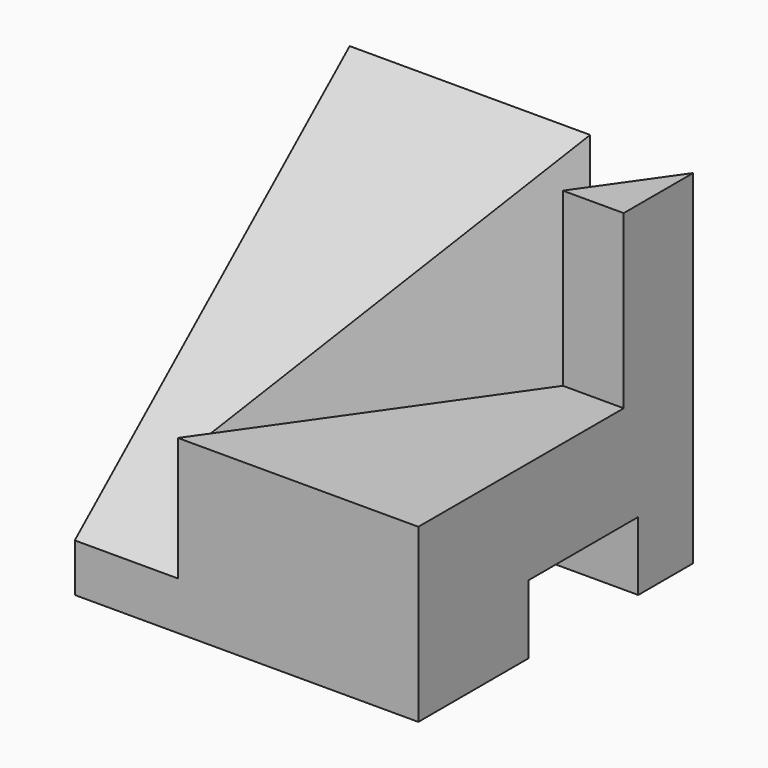
from build123d import *

# Parameters (mm, degrees)
F0_W      = 50
F0_H      = 50
F1_DEPTH  = 50
F3_DEPTH  = 43
F5_DEPTH  = 25
F8_REACH  = 113.7106781187
F10_DEPTH = 35
F12_REACH = 115.9479483752
F13_W     = 20
F13_H     = 10
F14_DEPTH = 30


with BuildPart() as f1:
    # F0 (on Front) → F1 (new body)
    with BuildSketch(Plane.XZ):
        with Locations((-25, 25)):
            Rectangle(F0_W, F0_H)
    extrude(amount=F1_DEPTH)

    # F2 (on face) → F3 (cut)
    with BuildSketch(Plane.XY.offset(50)):
        Polygon((-35, -50), (0, 0), (-50, 0), (-50, -50), align=None)
    extrude(amount=-F3_DEPTH, mode=Mode.SUBTRACT)

    # F4 (on face) → F5 (cut)
    with BuildSketch(Plane.XY.offset(50)):
        Polygon((0, -12.6445109037), (-8.8511576326, -12.6445109037), (-35, -50), (0, -50), align=None)
    extrude(amount=-F5_DEPTH, mode=Mode.SUBTRACT)

    f8_end = Plane(origin=(0, 0, 50), x_dir=(0, -0.8567360565, -0.515755106), z_dir=(0, 0.515755106, -0.8567360565))
    # F6 (on face) → F8 (join, up to a plane its end follows)
    with BuildSketch(Plane.XY.offset(7)):
        Polygon((-50, 0), (-50, -50), (-35, -50), (0, 0), align=None)
    f8_long = extrude(amount=F8_REACH, mode=Mode.PRIVATE)
    add(split(f8_long, bisect_by=f8_end, keep=Keep.TOP, mode=Mode.PRIVATE))

    # F9 (on face) → F10 (cut)
    with BuildSketch(Plane.XY.offset(50)):
        Polygon((-28, -40), (0, 0), (-15, 0), (-43, -40), align=None)
    extrude(amount=-F10_DEPTH, mode=Mode.SUBTRACT)

    f12_end = Plane(origin=(-33.023255814, -47.1760797342, 23.3), x_dir=(-0.5734623444, -0.8192319205, 0), z_dir=(-0.8192319205, 0.5734623444, 0))
    # F11 (on face) → F12 (cut, up to a plane its end follows)
    with BuildSketch(Plane(origin=(-50, 0, 0), x_dir=(0, -1, 0), z_dir=(-1, 0, 0))):
        Polygon((50, 19.9), (0, 50), (50, 7), align=None)
    f12_long = extrude(amount=-F12_REACH, mode=Mode.PRIVATE)
    add(split(f12_long, bisect_by=f12_end, keep=Keep.TOP, mode=Mode.PRIVATE), mode=Mode.SUBTRACT)

    # F13 (on face) → F14 (cut)
    with BuildSketch(Plane.YZ):
        with Locations((-20, 5)):
            Rectangle(F13_W, F13_H)
    extrude(amount=-F14_DEPTH, mode=Mode.SUBTRACT)


solid = f1.part
